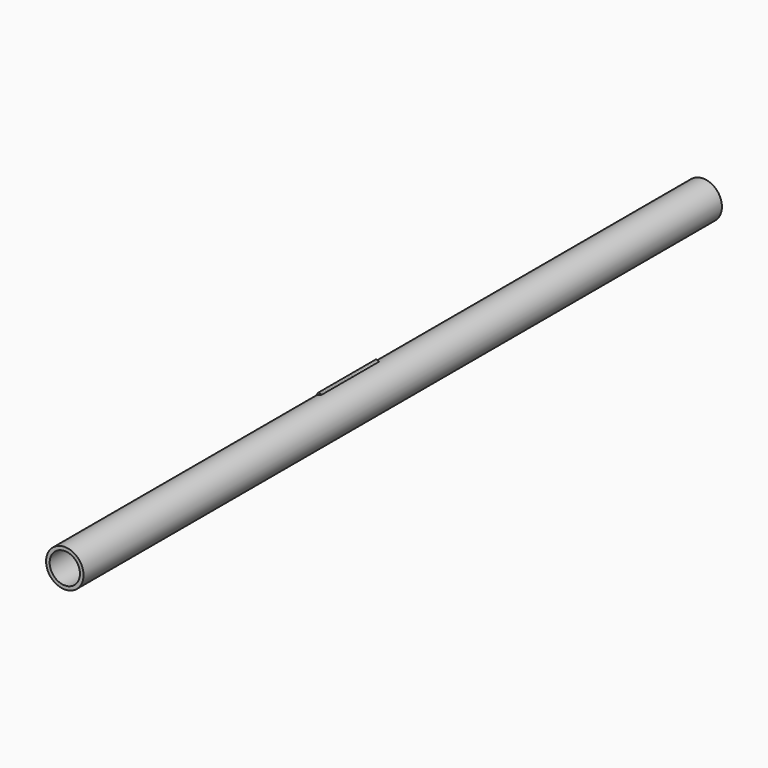
from build123d import *

# Parameters (mm, degrees)
F0_R      = 11.75
F0_R_2    = 9.5
F1_DEPTH  = 250
F3_DEPTH  = 6
F6_R      = 1
F8_DEPTH  = 20
F11_DEPTH = 25


# Not quite as in the source:
# - a feature of the source that left no trace in its solid (it failed there, or was rolled back) is left out


with BuildPart() as f1:
    # F0 (on Front) → F1 (new body, symmetric)
    with BuildSketch(Plane.XZ):
        Circle(F0_R)
        Circle(F0_R_2, mode=Mode.SUBTRACT)
    extrude(amount=F1_DEPTH, both=True)


with BuildPart() as f3:
    # F2 (on Front) → F3 (new body, symmetric)
    with BuildSketch(Plane.XZ):
        Polygon((9.3487489045, -12), (9.3487489045, 12), (-9.3487489045, 12), (-15.8130414784, 12), (-15.8130414784, 7.7571677975), (-9.3487489045, 3.5278871655), (-9.3487489045, -12), align=None)
    extrude(amount=F3_DEPTH, both=True)

    # F6
    f6_edges = [f3.edges().sort_by_distance(p)[0] for p in [
        (-12.580895, -6, 5.642527),
        (-15.813041, -6, 9.878584),
        (-3.232146, -6, 12),
        (9.348749, -6, 0),
        (0, -6, -12),
        (-9.348749, -6, -4.236056),
        (-12.580895, 6, 5.642527),
        (-9.348749, 6, -4.236056),
        (0, 6, -12),
        (9.348749, 6, 0),
        (-3.232146, 6, 12),
        (-15.813041, 6, 9.878584),
        (9.348749, 0, 12),
        (-15.813041, 0, 12),
        (-9.348749, 0, -12),
        (9.348749, 0, -12),
        (-15.813041, 0, 7.757168),
        (-9.348749, 0, 3.527887),
    ]]
    fillet(f6_edges, radius=F6_R)


with BuildPart() as f8:
    # F7 (on Front) → F8 (new body)
    with BuildSketch(Plane.XZ):
        with BuildLine():
            ThreePointArc((-1.3822059868, -7.8318203847), (-1.0457324806, -8.0702539027), (-0.6499857683, -8.1862258935))
            ThreePointArc((-0.6499857683, -8.1862258935), (0.6634160857, -7.3993051244), (0.2295820612, -5.9309534071))
            ThreePointArc((0.2295820612, -5.9309534071), (-1.659147278, -4.975633697), (-3.75, -4.6465909039))
            Line((-3.75, -4.6465909039), (-4.25, -4.6465909039))
            ThreePointArc((-4.25, -4.6465909039), (-5.25, 2.426704548), (-4.25, 9.5))
            ThreePointArc((-4.25, 9.5), (-3.6893800998, 9.837157335), (-3.3758418622, 10.411320652))
            ThreePointArc((-3.3758418622, 10.411320652), (-1.5633110072, 9.9380884638), (0.3087840895, 9.8711799181))
            ThreePointArc((0.3087840895, 9.8711799181), (2.6321750973, 9.7202080134), (1.0275972493, 11.4072966954))
            ThreePointArc((1.0275972493, 11.4072966954), (-1.5278224451, 10.9666658446), (-3.9849436446, 11.7954485495))
            ThreePointArc((-3.9849436446, 11.7954485495), (-5.669507399, 11.3351687839), (-5.25, 9.639991493))
            Line((-5.25, 9.639991493), (-10.8698996042, 5.7813227536))
            ThreePointArc((-10.8698996042, 5.7813227536), (-11.0586777654, 5.2035661447), (-10.5502594702, 4.8704734692))
            Line((-10.5502594702, 4.8704734692), (-6.1664506753, 4.5299796695))
            ThreePointArc((-6.1664506753, 4.5299796695), (-6.1226370951, -0.1690661794), (-5.25, -4.786582397))
            Line((-5.25, -4.786582397), (-12.7708408072, -5.3389740882))
            Line((-12.7708408072, -5.3389740882), (-12.5926968245, -7.7644134194))
            Line((-12.5926968245, -7.7644134194), (-11.1781490388, -7.6605175301))
            Line((-11.1781490388, -7.6605175301), (-4.0669947565, -7.1382165479))
            ThreePointArc((-4.0669947565, -7.1382165479), (-2.6675417013, -7.2641568314), (-1.3822059868, -7.8318203847))
        make_face()
    extrude(amount=F8_DEPTH)


with BuildPart() as f9_1:
    # F9: copy of F8
    add(f8.part)


with BuildPart() as f11:
    # F10 (on face) → F11 (new body)
    with BuildSketch(Plane.XZ.offset(20)):
        with BuildLine():
            ThreePointArc((-5.2538811343, -4.786867459), (-5.049711338, -5.5456859485), (-4.82626334, -6.2990529228))
            ThreePointArc((-4.82626334, -6.2990529228), (-4.5428267266, -6.8056736308), (-4.0669947565, -7.1382165479))
            ThreePointArc((-4.0669947565, -7.1382165479), (-3.6165429302, -7.1286492086), (-3.1675377255, -7.1659682104))
            ThreePointArc((-3.1675377255, -7.1659682104), (-2.2835624907, -5.8500557938), (-3.3303235399, -4.6595395152))
            ThreePointArc((-3.3303235399, -4.6595395152), (-3.5400619153, -4.6498288268), (-3.75, -4.6465909039))
            ThreePointArc((-3.75, -4.6465909039), (-4.0090231211, -4.7083857532), (-4.25, -4.821707086))
            ThreePointArc((-4.25, -4.821707086), (-5.2723597262, 2.339146457), (-4.25, 9.5))
            ThreePointArc((-4.25, 9.5), (-3.6893800998, 9.837157335), (-3.3758418622, 10.411320652))
            ThreePointArc((-3.3758418622, 10.411320652), (-1.5633110072, 9.9380884638), (0.3087840895, 9.8711799181))
            ThreePointArc((0.3087840895, 9.8711799181), (2.6321750973, 9.7202080134), (1.0275972493, 11.4072966954))
            ThreePointArc((1.0275972493, 11.4072966954), (0.9836866111, 11.3871083167), (0.9395874544, 11.3673351237))
            ThreePointArc((0.9395874544, 11.3673351237), (-1.4940307198, 10.9414868446), (-3.8439185328, 11.7042918268))
            ThreePointArc((-3.8439185328, 11.7042918268), (-3.914804649, 11.7492922671), (-3.9849436446, 11.7954485495))
            ThreePointArc((-3.9849436446, 11.7954485495), (-5.669507399, 11.3351687839), (-5.25, 9.639991493))
            Line((-5.25, 9.639991493), (-10.8698996042, 5.7813227536))
            ThreePointArc((-10.8698996042, 5.7813227536), (-11.0070885763, 5.2216701006), (-10.5502594702, 4.8704734692))
            Line((-10.5502594702, 4.8704734692), (-6.1664506753, 4.5299796695))
            ThreePointArc((-6.1664506753, 4.5299796695), (-6.0732938622, -0.087360616), (-5.291275385, -4.6389489768))
            ThreePointArc((-5.291275385, -4.6389489768), (-5.2707443813, -4.7127955149), (-5.25, -4.786582397))
            Line((-5.25, -4.786582397), (-5.2538811343, -4.786867459))
        make_face()
        with BuildLine():
            ThreePointArc((-3.1675377255, -7.1659682104), (-3.6165429302, -7.1286492086), (-4.0669947565, -7.1382165479))
            ThreePointArc((-4.0669947565, -7.1382165479), (-3.6197464137, -7.2324770688), (-3.1675377255, -7.1659682104))
        make_face()
    extrude(amount=F11_DEPTH)


solid = Compound([f1.part, f8.part, f9_1.part, f11.part])
